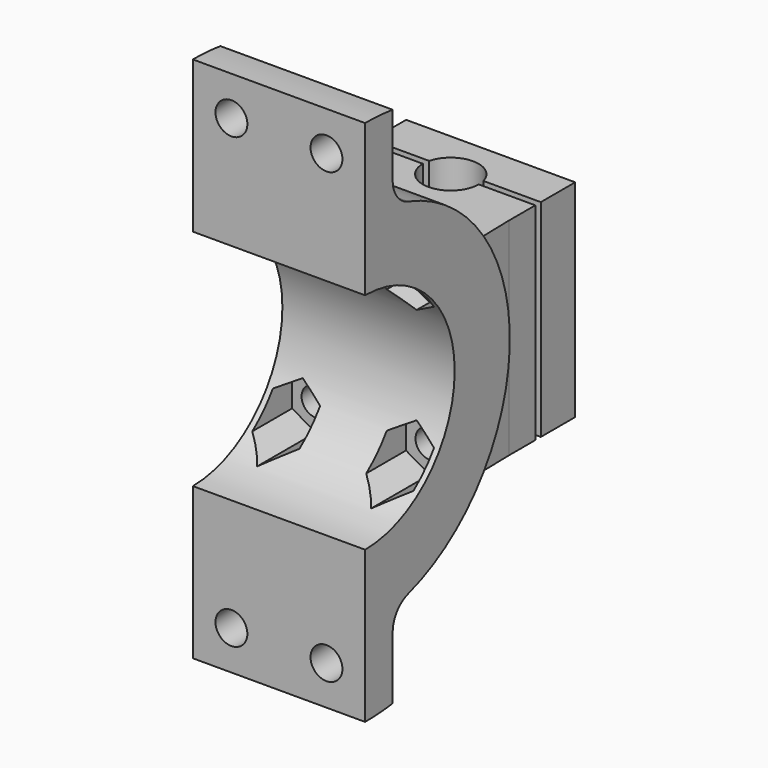
from build123d import *

# Parameters (mm, degrees)
F1_DEPTH  = 12.5
F2_R      = 2.3120560343
F3_DEPTH  = 26.251
F5_DEPTH  = 15
F6_R      = 2.05
F7_DEPTH  = 35
F9_R      = 2.05
F10_DEPTH = 25


# Not quite as in the source:
# - ends of sketch curves that miss each other by under 0.0002 mm in the source are joined


with BuildPart() as f1:
    # F0 (on Right) → F1 (new body, symmetric)
    with BuildSketch(Plane.YZ):
        with BuildLine():
            ThreePointArc((0, 16.25), (16.25, 0), (0, -16.25))
            Line((0, -16.25), (0, -38.25))
            ThreePointArc((0, -38.25), (2.5053801525, -38.1678604364), (5, -37.921794525))
            Line((5, -37.921794525), (4.9999998882, -28.8786509221))
            ThreePointArc((4.9999998882, -28.8786509221), (5.7778380649, -26.509152159), (7.8086833246, -25.0616632476))
            ThreePointArc((7.8086833246, -25.0616632476), (26.25, -5.08e-08), (7.8086834216, 25.0616632174))
            ThreePointArc((7.8086834216, 25.0616632174), (5.7778381721, 26.5091521304), (5, 28.8786508873))
            Line((5, 28.8786508873), (5, 37.921794525))
            ThreePointArc((5, 37.921794525), (2.5053801525, 38.1678604364), (0, 38.25))
            Line((0, 38.25), (0, 16.25))
        make_face()
    extrude(amount=F1_DEPTH, both=True)

    # F2 (on Front) → F3 (cut, through all)
    with BuildSketch(Plane.XZ):
        with Locations((6.896616891, 32.556977123)):
            Circle(F2_R)
        with Locations((-6.896616891, 32.556977123)):
            Circle(F2_R)
        with Locations((-6.896616891, -32.556977123)):
            Circle(F2_R)
        with Locations((6.896616891, -32.556977123)):
            Circle(F2_R)
    extrude(amount=-F3_DEPTH, mode=Mode.SUBTRACT)

    # F4 (on Top) → F5 (join, symmetric)
    with BuildSketch(Plane.XY):
        with BuildLine():
            ThreePointArc((4.05, 31.1641552804), (0, 27.1141552804), (-4.05, 31.1641552804))
            Line((-4.05, 31.1641552804), (-12.2654928641, 31.1641552804))
            Line((-12.2654928641, 31.1641552804), (-12.2654928641, 26.3486900835))
            Line((-12.2654928641, 26.3486900835), (-12.2654928641, 25.9208133907))
            Line((-12.2654928641, 25.9208133907), (-12.2654928641, 19.209831953))
            Line((-12.2654928641, 19.209831953), (-10.1258861735, 19.209831953))
            Line((-10.1258861735, 19.209831953), (10.1258861735, 19.209831953))
            Line((10.1258861735, 19.209831953), (12.4368978535, 19.209831953))
            Line((12.4368978535, 19.209831953), (12.2654928641, 26.3595975861))
            Line((12.2654928641, 26.3595975861), (12.2654928641, 31.1641552804))
            Line((12.2654928641, 31.1641552804), (4.05, 31.1641552804))
        make_face()
        with BuildLine():
            Line((-12.2654928641, 25.9208133907), (-12.2654928641, 26.3486900835))
            ThreePointArc((-12.2654928641, 26.3486900835), (-12.2673585101, 26.1347517371), (-12.2654928641, 25.9208133907))
        make_face()
    extrude(amount=F5_DEPTH, both=True)


with BuildPart() as f5:
    # F4 (on Top) → F5, piece 2 (new body, symmetric)
    with BuildSketch(Plane.XY):
        with BuildLine():
            Line((12.2654928641, 38.4021102472), (0, 38.4021102472))
            Line((0, 38.4021102472), (-12.2654928641, 38.4021102472))
            Line((-12.2654928641, 38.4021102472), (-12.2654928641, 32.1641552804))
            Line((-12.2654928641, 32.1641552804), (-3.9246018906, 32.1641552804))
            ThreePointArc((-3.9246018906, 32.1641552804), (0, 35.2141552804), (3.9246018906, 32.1641552804))
            Line((3.9246018906, 32.1641552804), (12.2654928641, 32.1641552804))
            Line((12.2654928641, 32.1641552804), (12.2654928641, 38.4021102472))
        make_face()
    extrude(amount=F5_DEPTH, both=True)


with BuildPart() as f7_tool:
    # F6 (on face) → F7 (new body)
    with BuildSketch(Plane(origin=(0, 38.4021102472, 0), x_dir=(-1, 0, 0), z_dir=(0, 1, 0))):
        with Locations((-8.2654928641, 11)):
            Circle(F6_R)
        with Locations((8.2654928641, 11)):
            Circle(F6_R)
        with Locations((-8.2654928641, -11)):
            Circle(F6_R)
        with Locations((8.2654928641, -11)):
            Circle(F6_R)
    extrude(amount=-F7_DEPTH)


with BuildPart() as f1_1:
    add(f1.part)

    # F7: cut by f7_tool
    add(f7_tool.part, mode=Mode.SUBTRACT)

    # F9 (on offset) → F10 (cut)
    with BuildSketch(Plane.XZ.offset(-17)):
        Polygon((4.8404928641, 12.977424672), (4.8404928641, 9.022575328), (8.2654928641, 7.0451506561), (11.6904928641, 9.022575328), (11.6904928641, 12.977424672), (8.2654928641, 14.9548493439), align=None)
        with Locations((8.2654928641, 11)):
            Circle(F9_R, mode=Mode.SUBTRACT)
        Polygon((-4.8404928641, 9.022575328), (-4.8404928641, 12.977424672), (-8.2654928641, 14.9548493439), (-11.6904928641, 12.977424672), (-11.6904928641, 9.022575328), (-8.2654928641, 7.0451506561), align=None)
        with Locations((-8.2654928641, 11)):
            Circle(F9_R, mode=Mode.SUBTRACT)
        Polygon((8.2654928641, -7.0451506561), (4.8404928641, -9.022575328), (4.8404928641, -12.977424672), (8.2654928641, -14.9548493439), (11.6904928641, -12.977424672), (11.6904928641, -9.022575328), align=None)
        with Locations((8.2654928641, -11)):
            Circle(F9_R, mode=Mode.SUBTRACT)
        Polygon((-11.6904928641, -9.022575328), (-11.6904928641, -12.977424672), (-8.2654928641, -14.9548493439), (-4.8404928641, -12.977424672), (-4.8404928641, -9.022575328), (-8.2654928641, -7.0451506561), align=None)
        with Locations((-8.2654928641, -11)):
            Circle(F9_R, mode=Mode.SUBTRACT)
    extrude(amount=F10_DEPTH, mode=Mode.SUBTRACT)


with BuildPart() as f5_1:
    add(f5.part)

    # F7: cut by f7_tool
    add(f7_tool.part, mode=Mode.SUBTRACT)


solid = Compound([f1_1.part, f5_1.part])
